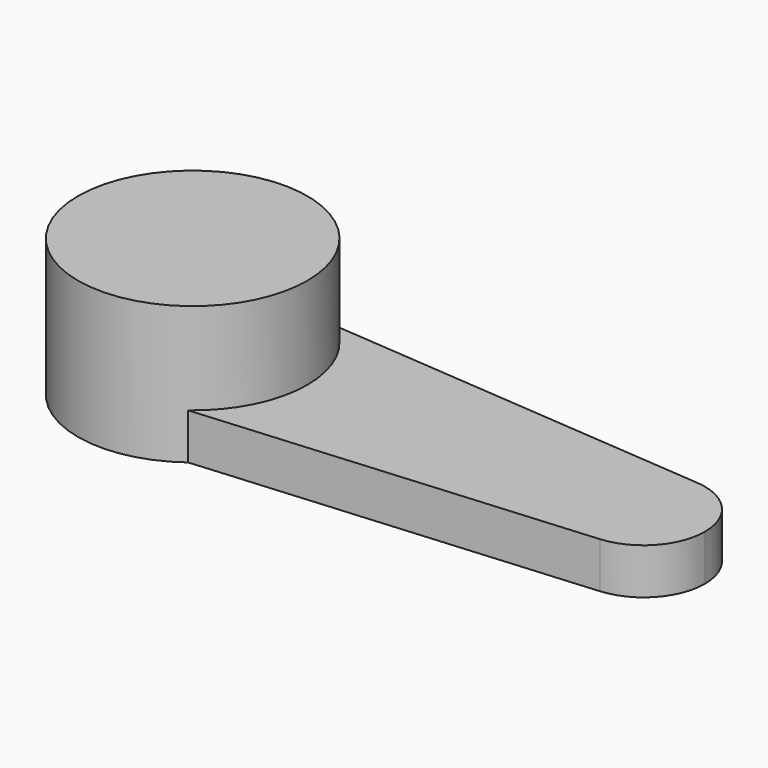
from build123d import *

# Parameters (mm, degrees)
F1_DEPTH = 1.5
F2_DEPTH = 4.5


# Not quite as in the source:
# - a feature names something its author has since deleted; it is built from what else it names


with BuildPart() as f1:
    # F0 (on Top) → F1 (new body)
    with BuildSketch(Plane.XY):
        with BuildLine():
            ThreePointArc((2.25, -3), (3.3541019662, -1.6770509831), (3.75, 0))
            ThreePointArc((3.75, 0), (3.3541019662, 1.6770509831), (2.25, 3))
            ThreePointArc((2.25, 3), (-3.75, 0), (2.25, -3))
        make_face()
        with BuildLine():
            ThreePointArc((16.75, 0), (16.2191802202, 1.3570222845), (14.9084905194, 1.9937102987))
            ThreePointArc((14.9084905194, 1.9937102987), (12.75, 0), (14.9084905194, -1.9937102987))
            ThreePointArc((14.9084905194, -1.9937102987), (16.2191802202, -1.3570222845), (16.75, 0))
        make_face()
        with BuildLine():
            ThreePointArc((2.25, 3), (3.3541019662, 1.6770509831), (3.75, 0))
            ThreePointArc((3.75, 0), (3.3541019662, -1.6770509831), (2.25, -3))
            Line((2.25, -3), (14.9084905194, -1.9937102987))
            ThreePointArc((14.9084905194, -1.9937102987), (12.75, 0), (14.9084905194, 1.9937102987))
            Line((14.9084905194, 1.9937102987), (2.25, 3))
        make_face()
    extrude(amount=F1_DEPTH)

    # F0 (on Top) → F2 (join)
    with BuildSketch(Plane.XY):
        with BuildLine():
            ThreePointArc((2.25, -3), (3.3541019662, -1.6770509831), (3.75, 0))
            ThreePointArc((3.75, 0), (3.3541019662, 1.6770509831), (2.25, 3))
            ThreePointArc((2.25, 3), (-3.75, 0), (2.25, -3))
        make_face()
    extrude(amount=F2_DEPTH)


solid = f1.part
